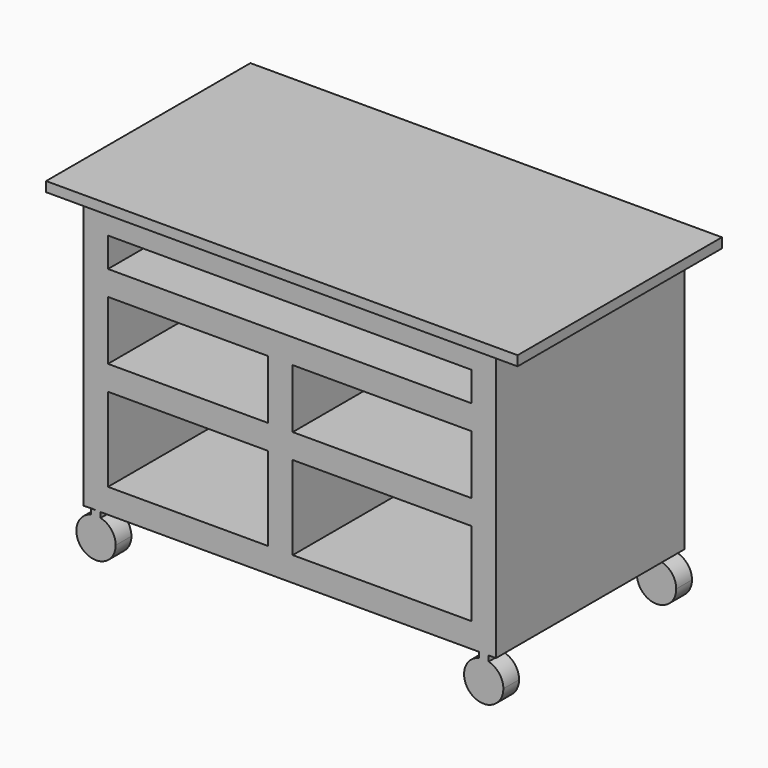
from build123d import *

# Parameters (mm, degrees)
F0_W     = 414.2166706732
F0_H     = 63.5
F0_W_2   = 63.5
F0_H_2   = 216.5272635669
F0_W_3   = 462.0833293268
F0_H_3   = 152.4
F1_DEPTH = 609.6
F2_DEPTH = 609.6
F5_DEPTH = 1242.06
F6_W     = 19.05
F6_H     = 699.1272635669
F7_DEPTH = 1066.8
F8_W     = 1219.2
F8_H     = 660.4
F8_W_2   = 1066.8
F8_H_2   = 609.6
F9_DEPTH = 25.4


with BuildPart() as f1:
    # F0 (on Front) → F1 (new body)
    with BuildSketch(Plane.XZ):
        Polygon((469.9, -273.3665645704), (469.9, -317.8136317834), (488.95, -317.8136317834), (488.95, -292.4136317834), (514.35, -292.4136317834), (514.35, -317.8136317834), (533.4, -317.8136317834), (533.4, 317.8136317834), (469.9, 317.8136317834), (469.9, 241.6136317834), (469.9, 178.1136317834), (469.9, 25.7136317834), (469.9, -37.7863682166), (469.9, -254.3136317834), align=None)
        Polygon((-469.9, -317.8136317834), (469.9, -317.8136317834), (469.9, -273.3665645704), (469.9, -254.3136317834), (7.8166706732, -254.3136317834), (-55.6833293268, -254.3136317834), (-469.9, -254.3136317834), align=None)
        Polygon((-488.9560716881, -317.8136317834), (-469.9, -317.8136317834), (-469.9, -254.3136317834), (-469.9, -37.7863682166), (-469.9, 25.7136317834), (-469.9, 178.1136317834), (-469.9, 241.6136317834), (-469.9, 317.8136317834), (-533.4, 317.8136317834), (-533.4, -317.8136317834), (-514.3560716881, -317.4411400029), (-514.3560716881, -291.792732976), (-488.9560716881, -291.792732976), align=None)
        Polygon((488.95, -292.4136317834), (488.95, -317.8136317834), (501.65, -317.8136317834), (514.35, -317.8136317834), (514.35, -292.4136317834), align=None)
        Polygon((-501.6472799932, -317.8136317834), (-488.9560716881, -317.8136317834), (-488.9560716881, -291.792732976), (-514.3560716881, -291.792732976), (-514.3560716881, -317.4411400029), (-501.6560716881, -317.192732976), align=None)
        with Locations((-262.7916646634, -6.0363682166)):
            Rectangle(F0_W, F0_H)
        with Locations((-23.9333293268, -146.05)):
            Rectangle(F0_W_2, F0_H_2)
        with Locations((238.8583353366, -6.0363682166)):
            Rectangle(F0_W_3, F0_H)
        with Locations((-23.9333293268, -6.0363682166)):
            Rectangle(F0_W_2, F0_H)
        Polygon((-469.9, 241.6136317834), (-469.9, 178.1136317834), (-55.6833293268, 178.1136317834), (7.8166706732, 178.1136317834), (469.9, 178.1136317834), (469.9, 241.6136317834), align=None)
        with Locations((-23.9333293268, 101.9136317834)):
            Rectangle(F0_W_2, F0_H_3)
        Polygon((469.9, 317.8136317834), (533.4, 317.8136317834), (533.4, 381.3136317834), (-533.4, 381.3136317834), (-533.4, 317.8136317834), (-469.9, 317.8136317834), align=None)
    extrude(amount=F1_DEPTH)

    # F0 (on Front) → F2 (join)
    with BuildSketch(Plane.XZ):
        with BuildLine():
            ThreePointArc((-449.9570255615, -380.6863682166), (-460.8814161194, -349.2129544898), (-488.9560716881, -331.2760708315))
            Line((-488.9560716881, -331.2760708315), (-488.9560716881, -342.592732976))
            Line((-488.9560716881, -342.592732976), (-501.2964171884, -342.592732976))
            Line((-501.2964171884, -342.592732976), (-514.3560716881, -342.592732976))
            Line((-514.3560716881, -342.592732976), (-514.3560716881, -331.7404190027))
            ThreePointArc((-514.3560716881, -331.7404190027), (-531.4963200945, -421.1305986038), (-449.9570255615, -380.6863682166))
        make_face()
        with BuildLine():
            Line((-501.2964171884, -342.592732976), (-501.4762624628, -329.8914600241))
            ThreePointArc((-501.4762624628, -329.8914600241), (-507.9756105712, -330.4018573762), (-514.3560716881, -331.7404190027))
            Line((-514.3560716881, -331.7404190027), (-514.3560716881, -342.592732976))
            Line((-514.3560716881, -342.592732976), (-501.2964171884, -342.592732976))
        make_face()
        with BuildLine():
            Line((-501.4762624628, -329.8914600241), (-501.6472799932, -317.8136317834))
            Line((-501.6472799932, -317.8136317834), (-514.3560716881, -317.8136317834))
            Line((-514.3560716881, -317.8136317834), (-514.3560716881, -331.7404190027))
            ThreePointArc((-514.3560716881, -331.7404190027), (-507.9756105712, -330.4018573762), (-501.4762624628, -329.8914600241))
        make_face()
        with BuildLine():
            Line((-488.9560716881, -331.2760708315), (-488.9560716881, -317.8136317834))
            Line((-488.9560716881, -317.8136317834), (-501.6472799932, -317.8136317834))
            Line((-501.6472799932, -317.8136317834), (-501.4762624628, -329.8914600241))
            ThreePointArc((-501.4762624628, -329.8914600241), (-495.1730843427, -330.194194561), (-488.9560716881, -331.2760708315))
        make_face()
        with BuildLine():
            Line((-488.9560716881, -342.592732976), (-488.9560716881, -331.2760708315))
            ThreePointArc((-488.9560716881, -331.2760708315), (-495.1730843427, -330.194194561), (-501.4762624628, -329.8914600241))
            Line((-501.4762624628, -329.8914600241), (-501.2964171884, -342.592732976))
            Line((-501.2964171884, -342.592732976), (-488.9560716881, -342.592732976))
        make_face()
        with BuildLine():
            Line((488.95, -343.2136317834), (488.95, -332.1267432866))
            ThreePointArc((488.95, -332.1267432866), (470.5414802667, -421.4745580676), (552.45, -381.3136317834))
            ThreePointArc((552.45, -381.3136317834), (541.8109262841, -350.2051120501), (514.35, -332.1267432866))
            Line((514.35, -332.1267432866), (514.35, -343.2136317834))
            Line((514.35, -343.2136317834), (501.65, -343.2136317834))
            Line((501.65, -343.2136317834), (488.95, -343.2136317834))
        make_face()
        with BuildLine():
            ThreePointArc((514.35, -332.1267432866), (508.0510180581, -330.9185232131), (501.65, -330.5136317834))
            Line((501.65, -330.5136317834), (501.65, -343.2136317834))
            Line((501.65, -343.2136317834), (514.35, -343.2136317834))
            Line((514.35, -343.2136317834), (514.35, -332.1267432866))
        make_face()
        with BuildLine():
            Line((501.65, -317.8136317834), (488.95, -317.8136317834))
            Line((488.95, -317.8136317834), (488.95, -332.1267432866))
            ThreePointArc((488.95, -332.1267432866), (495.2489819419, -330.9185232131), (501.65, -330.5136317834))
            Line((501.65, -330.5136317834), (501.65, -317.8136317834))
        make_face()
        with BuildLine():
            Line((514.35, -317.8136317834), (501.65, -317.8136317834))
            Line((501.65, -317.8136317834), (501.65, -330.5136317834))
            ThreePointArc((501.65, -330.5136317834), (508.0510180581, -330.9185232131), (514.35, -332.1267432866))
            Line((514.35, -332.1267432866), (514.35, -317.8136317834))
        make_face()
        with BuildLine():
            ThreePointArc((501.65, -330.5136317834), (495.2489819419, -330.9185232131), (488.95, -332.1267432866))
            Line((488.95, -332.1267432866), (488.95, -343.2136317834))
            Line((488.95, -343.2136317834), (501.65, -343.2136317834))
            Line((501.65, -343.2136317834), (501.65, -330.5136317834))
        make_face()
    extrude(amount=F2_DEPTH)

    # F4 (on offset) → F5 (cut)
    with BuildSketch(Plane.YZ.offset(660.4)):
        Polygon((-50.8, -317.8136317834), (-558.8, -317.8136317834), (-558.8, -353.9129836664), (-558.8, -456.8212373361), (-50.8, -456.8212373361), (-50.8, -353.9129836664), align=None)
    extrude(amount=-F5_DEPTH, mode=Mode.SUBTRACT)

    # F6 (on face) → F7 (join)
    with BuildSketch(Plane(origin=(-533.4, 0, 0), x_dir=(0, -1, 0), z_dir=(-1, 0, 0))):
        with Locations((9.525, 31.75)):
            Rectangle(F6_W, F6_H)
    extrude(amount=-F7_DEPTH)


with BuildPart() as f9:
    # F8 (on face) → F9 (new body)
    with BuildSketch(Plane.XY.offset(381.3136317834)):
        with Locations((0, -304.8)):
            Rectangle(F8_W, F8_H)
        with Locations((0, -304.8)):
            Rectangle(F8_W_2, F8_H_2, mode=Mode.SUBTRACT)
        with Locations((0, -304.8)):
            Rectangle(F8_W_2, F8_H_2)
    extrude(amount=F9_DEPTH)


solid = Compound([f1.part, f9.part])
